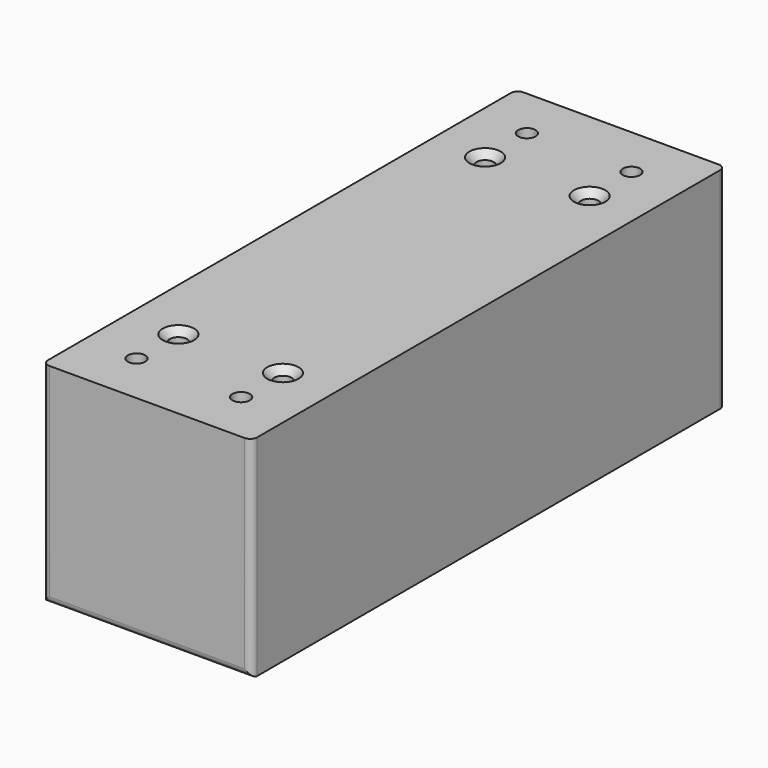
from build123d import *

# Parameters (mm, degrees)
F0_R     = 2.5
F1_DEPTH = 5
F2_W     = 170
F2_H     = 50.3
F3_DEPTH = 5
F4_W     = 55
F4_H     = 50.3
F5_DEPTH = 5
F7_R     = 2.5
F8_DEPTH = 5
F9_SIZE  = 2
F10_SIZE = 2
F11_SIZE = 2
F12_R    = 2


# Not quite as in the source:
# - a feature names something its author has since deleted; it is built from what else it names


with BuildPart() as f1:
    # F0 (on Top) → F1 (new body)
    with BuildSketch(Plane.XY):
        with BuildLine():
            Line((-60, 0), (0, 0))
            Line((0, 0), (0, 150))
            Line((0, 150), (0, 170))
            Line((0, 170), (-15, 170))
            add(Edge.make_bspline(
                [(-15, 170), (-14.4841735922, 160.0600889734), (-13.9683471845, 150.1201779469), (-13.6234299021, 140.3529161241)],
                knots=[0, 0, 0, 0, 0.0906883322, 0.0906883322, 0.0906883322, 0.0906883322], degree=3))
            add(Edge.make_bspline(
                [(-13.6234299021, 140.3529161241), (-12.0632834056, 96.1731661082), (-14.5980537911, 42.9711861088), (-50.2193379026, 23.1925838291), (-60, 19.9139873857)],
                knots=[0.0906883322, 0.0906883322, 0.0906883322, 0.0906883322, 0.5008941728, 0.6275927921, 0.6275927921, 0.6275927921, 0.6275927921], degree=3))
            Line((-60, 19.9139873857), (-60, 0))
        make_face()
        with Locations((-21.5087961406, 26.8674660474)):
            Circle(F0_R, mode=Mode.SUBTRACT)
        with BuildLine():
            ThreePointArc((-23.6172004723, 150), (-16.6720280929, 147.1947606368), (-13.6234299021, 140.3529161241))
            add(Edge.make_bspline(
                [(-15, 170), (-14.4841735922, 160.0600889734), (-13.9683471845, 150.1201779469), (-13.6234299021, 140.3529161241)],
                knots=[0, 0, 0, 0, 0.0906883322, 0.0906883322, 0.0906883322, 0.0906883322], degree=3))
            Line((-15, 170), (-25, 170))
            Line((-25, 170), (-25, 150))
            Line((-25, 150), (-23.6172004723, 150))
        make_face()
        with Locations((-18.0946737528, 160.0040644407)):
            Circle(F0_R, mode=Mode.SUBTRACT)
    extrude(amount=F1_DEPTH)

    # F2 (on face) → F3 (join)
    with BuildSketch(Plane.YZ):
        with Locations((85, 30.15)):
            Rectangle(F2_W, F2_H)
    extrude(amount=-F3_DEPTH)

    # F4 (on face) → F5 (join)
    with BuildSketch(Plane.XZ):
        with Locations((-32.5, 30.15)):
            Rectangle(F4_W, F4_H)
    extrude(amount=-F5_DEPTH)

    # F7 (on face) → F8 (join)
    with BuildSketch(Plane.XY.offset(55.3)):
        Polygon((-15, 0), (0, 0), (0, 15), (0, 155), (0, 170), (-15, 170), (-45, 170), (-60, 170), (-60, 155), (-60, 15), (-60, 0), (-45, 0), align=None)
        with Locations((-45, 15)):
            Circle(F7_R, mode=Mode.SUBTRACT)
        with Locations((-45, 30)):
            Circle(F7_R, mode=Mode.SUBTRACT)
        with Locations((-15, 15)):
            Circle(F7_R, mode=Mode.SUBTRACT)
        with Locations((-15, 30)):
            Circle(F7_R, mode=Mode.SUBTRACT)
        with Locations((-45, 140)):
            Circle(F7_R, mode=Mode.SUBTRACT)
        with Locations((-45, 155)):
            Circle(F7_R, mode=Mode.SUBTRACT)
        with Locations((-15, 140)):
            Circle(F7_R, mode=Mode.SUBTRACT)
        with Locations((-15, 155)):
            Circle(F7_R, mode=Mode.SUBTRACT)
    extrude(amount=F8_DEPTH)

    # F9
    f9_edges = [f1.edges().sort_by_distance(p)[0] for p in [
        (-17.5, 140, 60.3),
        (-47.5, 140, 60.3),
        (-17.5, 30, 60.3),
        (-47.5, 30, 60.3),
    ]]
    chamfer(f9_edges, length=F9_SIZE)

    # F10
    f10_edges = [f1.edges().sort_by_distance(p)[0] for p in [
        (-47.5, 155, 55.3),
        (-17.5, 155, 55.3),
        (-47.5, 15, 55.3),
        (-17.5, 15, 55.3),
    ]]
    chamfer(f10_edges, length=F10_SIZE)

    # F11
    f11_edges = [f1.edges().sort_by_distance(p)[0] for p in [
        (-24.008796, 26.867466, 0),
        (-20.594674, 160.004064, 0),
    ]]
    chamfer(f11_edges, length=F11_SIZE)

    # F12
    f12_edges = [f1.edges().sort_by_distance(p)[0] for p in [
        (0, 0, 30.15),
        (-60, 0, 30.15),
        (-30, 0, 0),
        (0, 170, 30.15),
        (-60, 170, 57.8),
    ]]
    fillet(f12_edges, radius=F12_R)


solid = f1.part
